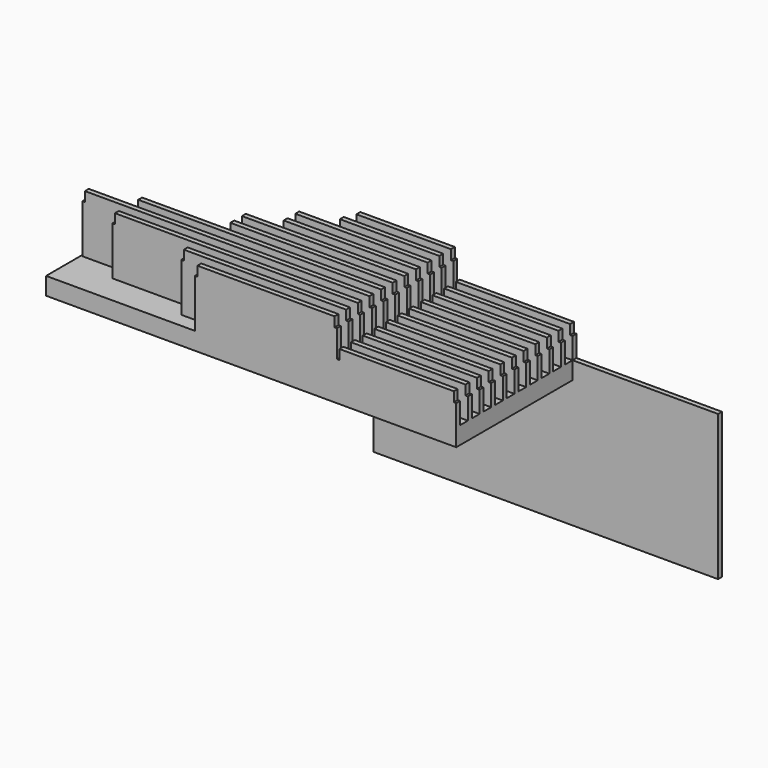
from build123d import *

# Parameters (mm, degrees)
F1_DEPTH  = 123
F2_DEPTH  = 300
F3_R      = 0.5
F4_DEPTH  = 1
F5_W      = 123
F5_H      = 28
F6_DEPTH  = 300
F7_W      = 2.5
F7_H      = 10
F8_DEPTH  = 300
F9_W      = 150
F9_H      = 150
F10_DEPTH = 5
F11_W     = 5
F11_H     = 60
F12_DEPTH = 197.5
F13_W     = 20
F13_H     = 60
F14_DEPTH = 158.5
F15_W     = 20
F15_H     = 60
F15_W_2   = 5
F16_DEPTH = 127.5
F17_W     = 5
F17_H     = 60
F18_DEPTH = 44.5
F19_W     = 5
F19_H     = 60
F20_DEPTH = 1.5
F21_W     = 5
F21_H     = 60
F22_DEPTH = 153.5
F23_W     = 5
F23_H     = 10
F24_DEPTH = 2.5
F25_W     = 5
F25_H     = 10
F26_DEPTH = 2.5
F27_W     = 5
F27_H     = 10
F28_DEPTH = 2.5
F29_W     = 5
F29_H     = 10
F30_DEPTH = 2.5
F31_W     = 5
F31_H     = 10
F32_DEPTH = 2.5
F33_W     = 5
F33_H     = 10
F34_DEPTH = 2.5
F35_W     = 5
F35_H     = 10
F36_DEPTH = 2.5
F37_W     = 5
F37_H     = 10
F38_DEPTH = 2.5
F39_W     = 5
F39_H     = 10
F40_DEPTH = 2.5
F41_W     = 5
F41_H     = 10
F42_DEPTH = 2.5
F43_W     = 5
F43_H     = 10
F44_DEPTH = 2.5
F45_W     = 217.5729006529
F45_H     = 131.9425046444
F46_DEPTH = 5


# Not quite as in the source:
# - a feature names something its author has since deleted; it is built from what else it names


with BuildPart() as f1:
    # F0 (on Right) → F1 (new body)
    with BuildSketch(Plane.YZ):
        Polygon((179.2768240368, 60), (174.2768240368, 60), (174.2768240368, -18.0574953556), (324.2768240368, -18.0574953556), (324.2768240368, -150), (329.2768240368, -150), (329.2768240368, 60), (324.2768240368, 60), (324.2768240368, 0), (314.2768240368, 0), (314.2768240368, 60), (309.2768240368, 60), (309.2768240368, 0), (299.2768240368, 0), (299.2768240368, 60), (294.2768240368, 60), (294.2768240368, 0), (284.2768240368, 0), (284.2768240368, 60), (279.2768240368, 60), (279.2768240368, 0), (269.2768240368, 0), (269.2768240368, 60), (264.2768240368, 60), (264.2768240368, 0), (254.2768240368, 0), (254.2768240368, 60), (249.2768240368, 60), (249.2768240368, 0), (239.2768240368, 0), (239.2768240368, 60), (234.2768240368, 60), (234.2768240368, 0), (224.2768240368, 0), (224.2768240368, 60), (219.2768240368, 60), (219.2768240368, 0), (209.2768240368, 0), (209.2768240368, 60), (204.2768240368, 60), (204.2768240368, 0), (194.2768240368, 0), (194.2768240368, 60), (189.2768240368, 60), (189.2768240368, 0), (179.2768240368, 0), align=None)
    extrude(amount=F1_DEPTH)

    # F0 (on Right) → F2 (join)
    with BuildSketch(Plane.YZ):
        Polygon((179.2768240368, 60), (174.2768240368, 60), (174.2768240368, -18.0574953556), (324.2768240368, -18.0574953556), (324.2768240368, -150), (329.2768240368, -150), (329.2768240368, 60), (324.2768240368, 60), (324.2768240368, 0), (314.2768240368, 0), (314.2768240368, 60), (309.2768240368, 60), (309.2768240368, 0), (299.2768240368, 0), (299.2768240368, 60), (294.2768240368, 60), (294.2768240368, 0), (284.2768240368, 0), (284.2768240368, 60), (279.2768240368, 60), (279.2768240368, 0), (269.2768240368, 0), (269.2768240368, 60), (264.2768240368, 60), (264.2768240368, 0), (254.2768240368, 0), (254.2768240368, 60), (249.2768240368, 60), (249.2768240368, 0), (239.2768240368, 0), (239.2768240368, 60), (234.2768240368, 60), (234.2768240368, 0), (224.2768240368, 0), (224.2768240368, 60), (219.2768240368, 60), (219.2768240368, 0), (209.2768240368, 0), (209.2768240368, 60), (204.2768240368, 60), (204.2768240368, 0), (194.2768240368, 0), (194.2768240368, 60), (189.2768240368, 60), (189.2768240368, 0), (179.2768240368, 0), align=None)
    extrude(amount=-F2_DEPTH)

    # F3 (on face) → F4, piece 2 (join)
    with BuildSketch(Plane(origin=(0, 329.2768240368, 0), x_dir=(-1, 0, 0), z_dir=(0, 1, 0))):
        with Locations((-82.5385674834, -48.5965646803)):
            Circle(F3_R)
        with Locations((31.1017241329, -28.6999493837)):
            Circle(F3_R)
    extrude(amount=F4_DEPTH)

    # F5 (on face) → F6 (cut)
    with BuildSketch(Plane(origin=(0, 329.2768240368, 0), x_dir=(-1, 0, 0), z_dir=(0, 1, 0))):
        with Locations((-61.5, 46)):
            Rectangle(F5_W, F5_H)
    extrude(amount=-F6_DEPTH, mode=Mode.SUBTRACT)

    # F7 (on face) → F8 (cut)
    with BuildSketch(Plane(origin=(0, 329.2768240368, 0), x_dir=(-1, 0, 0), z_dir=(0, 1, 0))):
        with Locations((-1.25, 27)):
            Rectangle(F7_W, F7_H)
        with Locations((1.25, 55)):
            Rectangle(F7_W, F7_H)
        with Locations((-121.75, 27)):
            Rectangle(F7_W, F7_H)
    extrude(amount=-F8_DEPTH, mode=Mode.SUBTRACT)



with BuildPart() as f4:
    # F3 (on face) → F4 (new body)
    with BuildSketch(Plane(origin=(0, 329.2768240368, 0), x_dir=(-1, 0, 0), z_dir=(0, 1, 0))):
        with Locations((-203.3374607563, -30)):
            Circle(F3_R)
    extrude(amount=F4_DEPTH)


with BuildPart() as f1_1:
    add(f1.part)

    add(f4.part)  # F10 merges F4
    # F9 (on face) → F10 (join)
    with BuildSketch(Plane(origin=(0, 329.2768240368, 0), x_dir=(-1, 0, 0), z_dir=(0, 1, 0))):
        with Locations((-198, -75)):
            Rectangle(F9_W, F9_H)
    extrude(amount=-F10_DEPTH)

    # F11 (on face) → F12 (cut)
    with BuildSketch(Plane(origin=(-300, 0, 0), x_dir=(0, -1, 0), z_dir=(-1, 0, 0))):
        with Locations((-326.7768240368, 30)):
            Rectangle(F11_W, F11_H)
        with Locations((-311.7768240368, 30)):
            Rectangle(F11_W, F11_H)
    extrude(amount=-F12_DEPTH, mode=Mode.SUBTRACT)

    # F13 (on face) → F14 (cut)
    with BuildSketch(Plane(origin=(-300, 0, 0), x_dir=(0, -1, 0), z_dir=(-1, 0, 0))):
        with Locations((-289.2768240368, 30)):
            Rectangle(F13_W, F13_H)
    extrude(amount=-F14_DEPTH, mode=Mode.SUBTRACT)

    # F15 (on face) → F16 (cut)
    with BuildSketch(Plane(origin=(-300, 0, 0), x_dir=(0, -1, 0), z_dir=(-1, 0, 0))):
        with Locations((-259.2768240368, 30)):
            Rectangle(F15_W, F15_H)
        with Locations((-191.7768240368, 30)):
            Rectangle(F15_W_2, F15_H)
    extrude(amount=-F16_DEPTH, mode=Mode.SUBTRACT)

    # F17 (on face) → F18 (cut)
    with BuildSketch(Plane(origin=(-300, 0, 0), x_dir=(0, -1, 0), z_dir=(-1, 0, 0))):
        with Locations((-236.7768240368, 30)):
            Rectangle(F17_W, F17_H)
        with Locations((-206.7768240368, 30)):
            Rectangle(F17_W, F17_H)
    extrude(amount=-F18_DEPTH, mode=Mode.SUBTRACT)

    # F19 (on face) → F20 (cut)
    with BuildSketch(Plane(origin=(-300, 0, 0), x_dir=(0, -1, 0), z_dir=(-1, 0, 0))):
        with Locations((-221.7768240368, 30)):
            Rectangle(F19_W, F19_H)
    extrude(amount=-F20_DEPTH, mode=Mode.SUBTRACT)

    # F21 (on face) → F22 (cut)
    with BuildSketch(Plane(origin=(-300, 0, 0), x_dir=(0, -1, 0), z_dir=(-1, 0, 0))):
        with Locations((-176.7768240368, 30)):
            Rectangle(F21_W, F21_H)
    extrude(amount=-F22_DEPTH, mode=Mode.SUBTRACT)

    # F23 (on face) → F24 (cut)
    with BuildSketch(Plane(origin=(-298.5, 0, 0), x_dir=(0, -1, 0), z_dir=(-1, 0, 0))):
        with Locations((-221.7768240368, 55)):
            Rectangle(F23_W, F23_H)
    extrude(amount=-F24_DEPTH, mode=Mode.SUBTRACT)

    # F25 (on face) → F26 (cut)
    with BuildSketch(Plane(origin=(-255.5, 0, 0), x_dir=(0, -1, 0), z_dir=(-1, 0, 0))):
        with Locations((-236.7768240368, 55)):
            Rectangle(F25_W, F25_H)
    extrude(amount=-F26_DEPTH, mode=Mode.SUBTRACT)

    # F27 (on face) → F28 (cut)
    with BuildSketch(Plane(origin=(-255.5, 0, 0), x_dir=(0, -1, 0), z_dir=(-1, 0, 0))):
        with Locations((-206.7768240368, 55)):
            Rectangle(F27_W, F27_H)
    extrude(amount=-F28_DEPTH, mode=Mode.SUBTRACT)

    # F29 (on face) → F30 (cut)
    with BuildSketch(Plane(origin=(-172.5, 0, 0), x_dir=(0, -1, 0), z_dir=(-1, 0, 0))):
        with Locations((-251.7768240368, 55)):
            Rectangle(F29_W, F29_H)
    extrude(amount=-F30_DEPTH, mode=Mode.SUBTRACT)

    # F31 (on face) → F32 (cut)
    with BuildSketch(Plane(origin=(-172.5, 0, 0), x_dir=(0, -1, 0), z_dir=(-1, 0, 0))):
        with Locations((-191.7768240368, 55)):
            Rectangle(F31_W, F31_H)
    extrude(amount=-F32_DEPTH, mode=Mode.SUBTRACT)

    # F33 (on face) → F34 (cut)
    with BuildSketch(Plane(origin=(-172.5, 0, 0), x_dir=(0, -1, 0), z_dir=(-1, 0, 0))):
        with Locations((-266.7768240368, 55)):
            Rectangle(F33_W, F33_H)
    extrude(amount=-F34_DEPTH, mode=Mode.SUBTRACT)

    # F35 (on face) → F36 (cut)
    with BuildSketch(Plane(origin=(-146.5, 0, 0), x_dir=(0, -1, 0), z_dir=(-1, 0, 0))):
        with Locations((-176.7768240368, 55)):
            Rectangle(F35_W, F35_H)
    extrude(amount=-F36_DEPTH, mode=Mode.SUBTRACT)

    # F37 (on face) → F38 (cut)
    with BuildSketch(Plane(origin=(-141.5, 0, 0), x_dir=(0, -1, 0), z_dir=(-1, 0, 0))):
        with Locations((-281.7768240368, 55)):
            Rectangle(F37_W, F37_H)
    extrude(amount=-F38_DEPTH, mode=Mode.SUBTRACT)

    # F39 (on face) → F40 (cut)
    with BuildSketch(Plane(origin=(-141.5, 0, 0), x_dir=(0, -1, 0), z_dir=(-1, 0, 0))):
        with Locations((-296.7768240368, 55)):
            Rectangle(F39_W, F39_H)
    extrude(amount=-F40_DEPTH, mode=Mode.SUBTRACT)

    # F41 (on face) → F42 (join)
    with BuildSketch(Plane(origin=(-102.5, 0, 0), x_dir=(0, -1, 0), z_dir=(-1, 0, 0))):
        with Locations((-311.7768240368, 55)):
            Rectangle(F41_W, F41_H)
    extrude(amount=F42_DEPTH)

    # F43 (on face) → F44 (cut)
    with BuildSketch(Plane(origin=(-102.5, 0, 0), x_dir=(0, -1, 0), z_dir=(-1, 0, 0))):
        with Locations((-326.7768240368, 55)):
            Rectangle(F43_W, F43_H)
    extrude(amount=-F44_DEPTH, mode=Mode.SUBTRACT)

    # F45 (on face) → F46 (cut)
    with BuildSketch(Plane(origin=(0, 329.2768240368, 0), x_dir=(-1, 0, 0), z_dir=(0, 1, 0))):
        with Locations((191.2135496736, -84.0287476778)):
            Rectangle(F45_W, F45_H)
    extrude(amount=-F46_DEPTH, mode=Mode.SUBTRACT)


solid = f1_1.part
